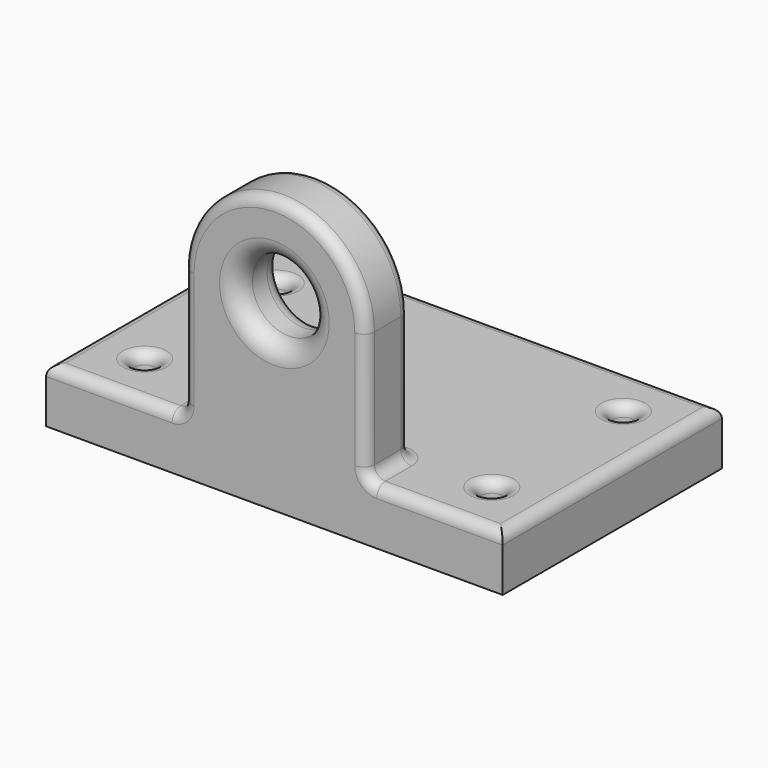
from build123d import *

# Parameters (mm, degrees)
F0_W     = 125
F0_H     = 75
F1_DEPTH = 15
F3_DEPTH = 15
F4_R     = 3
F5_DEPTH = 75.001
F6_R     = 3
F7_R     = 5


with BuildPart() as f1:
    # F0 (on Top) → F1 (new body)
    with BuildSketch(Plane.XY):
        Rectangle(F0_W, F0_H)
    extrude(amount=F1_DEPTH)

    # F2 (on face) → F3 (join)
    with BuildSketch(Plane.XZ.offset(37.5)):
        with BuildLine():
            Line((10, 50), (25, 50))
            ThreePointArc((25, 50), (0, 75), (-25, 50))
            Line((-25, 50), (-10, 50))
            ThreePointArc((-10, 50), (0, 60), (10, 50))
        make_face()
        with BuildLine():
            ThreePointArc((-25, 50), (0, 25), (25, 50))
            Line((25, 50), (10, 50))
            ThreePointArc((10, 50), (0, 40), (-10, 50))
            Line((-10, 50), (-25, 50))
        make_face()
        with BuildLine():
            Line((25, 15), (25, 50))
            ThreePointArc((25, 50), (0, 25), (-25, 50))
            Line((-25, 50), (-25, 15))
            Line((-25, 15), (25, 15))
        make_face()
    extrude(amount=-F3_DEPTH)

    # F4 (on face) → F5 (cut, through all)
    with BuildSketch(Plane(origin=(0, 0, 0), x_dir=(1, 0, 0), z_dir=(0, 0, -1))):
        with Locations((-47.5, 22.5)):
            Circle(F4_R)
        with Locations((47.5, 22.5)):
            Circle(F4_R)
        with Locations((47.5, -22.5)):
            Circle(F4_R)
        with Locations((-47.5, -22.5)):
            Circle(F4_R)
    extrude(amount=-F5_DEPTH, mode=Mode.SUBTRACT)

    # F6
    f6_edges = [f1.edges().sort_by_distance(p)[0] for p in [
        (0, -37.5, 75),
        (0, -22.5, 75),
        (25, -22.5, 32.5),
        (25, -37.5, 32.5),
        (-25, -37.5, 32.5),
        (-43.75, -37.5, 15),
        (-62.5, 0, 15),
        (0, 37.5, 15),
        (62.5, 0, 15),
        (43.75, -37.5, 15),
        (25, -30, 15),
        (-25, -30, 15),
        (-50.5, 22.5, 15),
        (-50.5, -22.5, 15),
        (44.5, -22.5, 15),
        (44.5, 22.5, 15),
        (0, -22.5, 15),
        (-25, -22.5, 32.5),
    ]]
    fillet(f6_edges, radius=F6_R)

    # F7
    f7_edges = [f1.edges().sort_by_distance(p)[0] for p in [
        (-10, -37.5, 50),
        (-10, -22.5, 50),
    ]]
    fillet(f7_edges, radius=F7_R)


solid = f1.part
